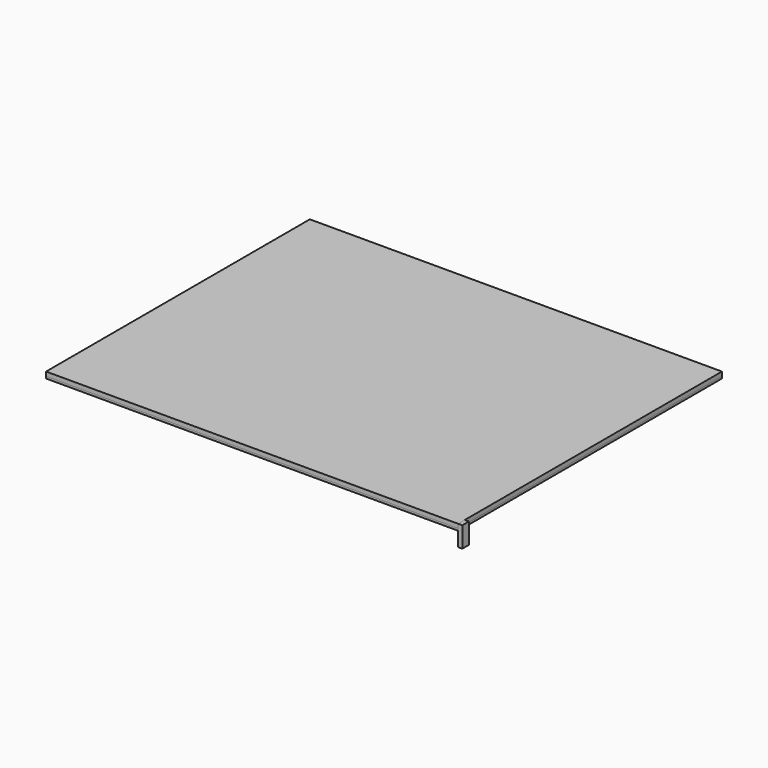
from build123d import *

# Parameters (mm, degrees)
F0_W     = 840
F0_H     = 80
F0_H_2   = 640
F1_DEPTH = 10
F2_DEPTH = 5
F3_W     = 20
F3_H     = 50
F4_DEPTH = 10


# Not quite as in the source:
# - a feature names something its author has since deleted; it is built from what else it names


with BuildPart() as f1:
    # F0 (on Top) → F1 (new body)
    with BuildSketch(Plane.XY):
        Polygon((-446.064549312, 490.2843640471), (-446.064549312, -309.7156359529), (-366.064549312, -309.7156359529), (-366.064549312, -229.7156359529), (-366.064549312, 410.2843640471), (-366.064549312, 490.2843640471), align=None)
        with Locations((53.935450688, -269.7156359529)):
            Rectangle(F0_W, F0_H)
        Polygon((473.935450688, -229.7156359529), (473.935450688, -309.7156359529), (553.935450688, -309.7156359529), (553.935450688, 490.2843640471), (473.935450688, 490.2843640471), (473.935450688, 410.2843640471), align=None)
        with Locations((53.935450688, 90.2843640471)):
            Rectangle(F0_W, F0_H_2)
        with Locations((53.935450688, 450.2843640471)):
            Rectangle(F0_W, F0_H)
    extrude(amount=F1_DEPTH)


with BuildPart() as f2:
    # F0 (on Top) → F2 (new body)
    with BuildSketch(Plane.XY):
        Polygon((-446.064549312, 490.2843640471), (-446.064549312, -309.7156359529), (-366.064549312, -309.7156359529), (-366.064549312, -229.7156359529), (-366.064549312, 410.2843640471), (-366.064549312, 490.2843640471), align=None)
        with Locations((53.935450688, 450.2843640471)):
            Rectangle(F0_W, F0_H)
        with Locations((53.935450688, -269.7156359529)):
            Rectangle(F0_W, F0_H)
        Polygon((473.935450688, -229.7156359529), (473.935450688, -309.7156359529), (553.935450688, -309.7156359529), (553.935450688, 490.2843640471), (473.935450688, 490.2843640471), (473.935450688, 410.2843640471), align=None)
    extrude(amount=-F2_DEPTH)


with BuildPart() as f4:
    # F3 (on face) → F4 (new body)
    with BuildSketch(Plane.YZ.offset(553.935450688)):
        with Locations((-299.7156359529, -15)):
            Rectangle(F3_W, F3_H)
    extrude(amount=F4_DEPTH)


solid = Compound([f1.part, f2.part, f4.part])
